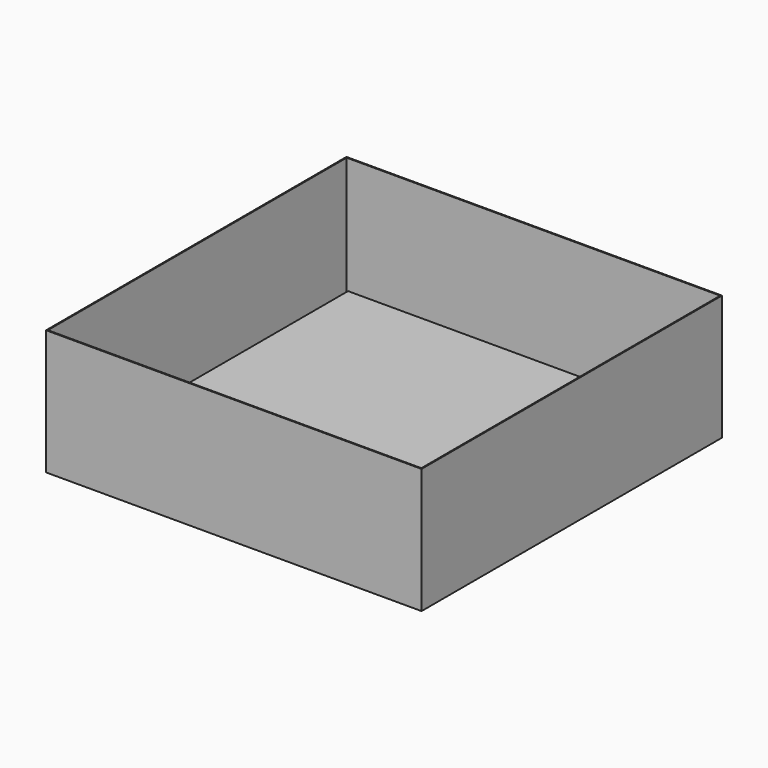
from build123d import *

# Parameters (mm, degrees)
F0_W     = 584.2
F0_H     = 584.2
F1_DEPTH = 19.05
F3_W     = 609.6
F3_H     = 609.6
F4_DEPTH = 203.2
F5_W     = 606.425
F5_H     = 606.425
F6_DEPTH = 201.6125


with BuildPart() as f1:
    # F0 (on Top) → F1 (new body)
    with BuildSketch(Plane.XY):
        Rectangle(F0_W, F0_H)
    extrude(amount=F1_DEPTH)


with BuildPart() as f4:
    # F3 (on offset) → F4 (new body)
    with BuildSketch(Plane(origin=(0, 0, -1.5875), x_dir=(1, 0, 0), z_dir=(0, 0, -1))):
        Rectangle(F3_W, F3_H)
    extrude(amount=-F4_DEPTH)

    # F5 (on face) → F6 (cut, through all)
    with BuildSketch(Plane.XY.offset(201.6125)):
        Rectangle(F5_W, F5_H)
    extrude(amount=-F6_DEPTH, mode=Mode.SUBTRACT)


solid = Compound([f1.part, f4.part])
